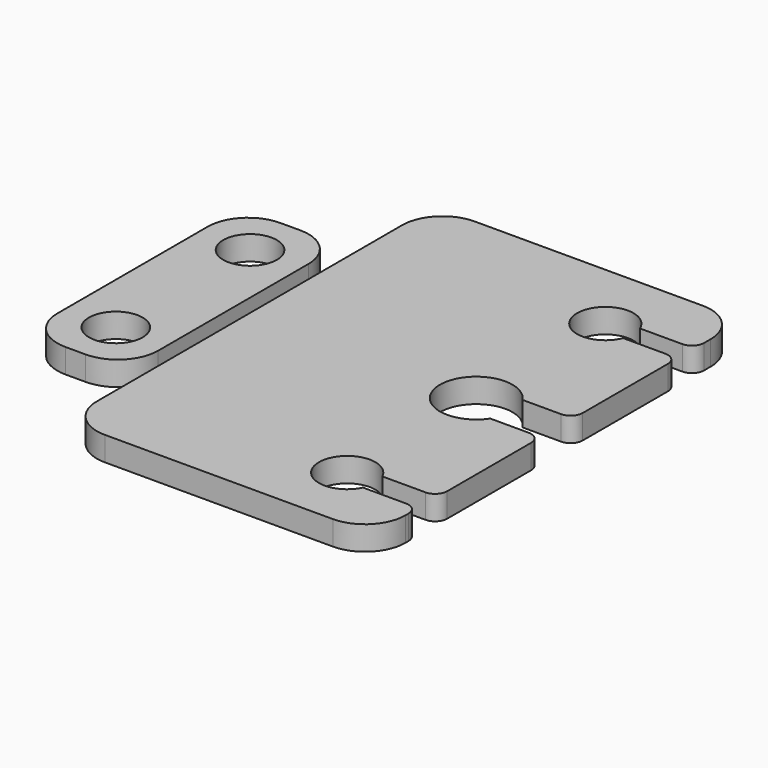
from build123d import *

# Parameters (mm, degrees)
F0_R     = 3.25
F1_DEPTH = 3
F2_R     = 5
F3_DEPTH = 5
F0_R_2   = 3.325
F4_DEPTH = 3
F5_R     = 5
F6_R     = 1.5


with BuildPart() as f1:
    # F0 (on Top) → F1 (new body)
    with BuildSketch(Plane.XY):
        with BuildLine():
            Line((-8.25, 28.8223753949), (-8.25, -28.4776246051))
            Line((-8.25, -28.4776246051), (30, -28.4776246051))
            Line((30, -28.4776246051), (30, -21.5))
            Line((30, -21.5), (23.1622776602, -21.5))
            ThreePointArc((23.1622776602, -21.5), (16.5, -20), (23.1622776602, -18.5))
            Line((23.1622776602, -18.5), (30, -18.5))
            Line((30, -18.5), (30, -2.5))
            Line((30, -2.5), (23.7416573868, -2.5))
            ThreePointArc((23.7416573868, -2.5), (15.5, 0), (23.7416573868, 2.5))
            Line((23.7416573868, 2.5), (30, 2.5))
            Line((30, 2.5), (30, 18.7))
            Line((30, 18.7), (23.2496153619, 18.7))
            ThreePointArc((23.2496153619, 18.7), (16.5, 20), (23.2496153619, 21.3))
            Line((23.2496153619, 21.3), (30, 21.3))
            Line((30, 21.3), (30, 28.8223753949))
            Line((30, 28.8223753949), (-8.25, 28.8223753949))
        make_face()
        with Locations((0, -10.2276246051)):
            Circle(F0_R, mode=Mode.SUBTRACT)
        with Locations((0, 10.5723753949)):
            Circle(F0_R, mode=Mode.SUBTRACT)
        with Locations((0, 10.5723753949)):
            Circle(F0_R)
        with Locations((0, -10.2276246051)):
            Circle(F0_R)
    extrude(amount=F1_DEPTH)

    # F2
    f2_edges = [f1.edges().sort_by_distance(p)[0] for p in [
        (-8.25, 28.822375, 1.5),
        (-8.25, -28.477625, 1.5),
        (30, -28.477625, 1.5),
        (30, 28.822375, 1.5),
    ]]
    fillet(f2_edges, radius=F2_R)

    # F0 (on Top) → F3 (join)
    with BuildSketch(Plane.XY):
        with Locations((0, 10.5723753949)):
            Circle(F0_R)
        with Locations((0, -10.2276246051)):
            Circle(F0_R)
    extrude(amount=-F3_DEPTH)

    # F6
    f6_edges = [f1.edges().sort_by_distance(p)[0] for p in [
        (30, -2.5, 1.5),
        (30, 2.5, 1.5),
        (30, 18.7, 1.5),
        (30, 21.3, 1.5),
        (30, -21.5, 1.5),
        (30, -18.5, 1.5),
    ]]
    fillet(f6_edges, radius=F6_R)


with BuildPart() as f4:
    # F0 (on Top) → F4 (new body)
    with BuildSketch(Plane.XY):
        Polygon((-10.25, 16.8223753949), (-16.5, 16.8223753949), (-22.75, 16.8223753949), (-22.75, -16.4776246051), (-16.5, -16.4776246051), (-10.25, -16.4776246051), align=None)
        with Locations((-16.5, -10.2276246051)):
            Circle(F0_R_2, mode=Mode.SUBTRACT)
        with Locations((-16.5, 10.5723753949)):
            Circle(F0_R_2, mode=Mode.SUBTRACT)
    extrude(amount=F4_DEPTH)

    # F5
    f5_edges = [f4.edges().sort_by_distance(p)[0] for p in [
        (-22.75, 16.822375, 1.5),
        (-22.75, -16.477625, 1.5),
        (-10.25, 16.822375, 1.5),
        (-10.25, -16.477625, 1.5),
    ]]
    fillet(f5_edges, radius=F5_R)


solid = Compound([f1.part, f4.part])
